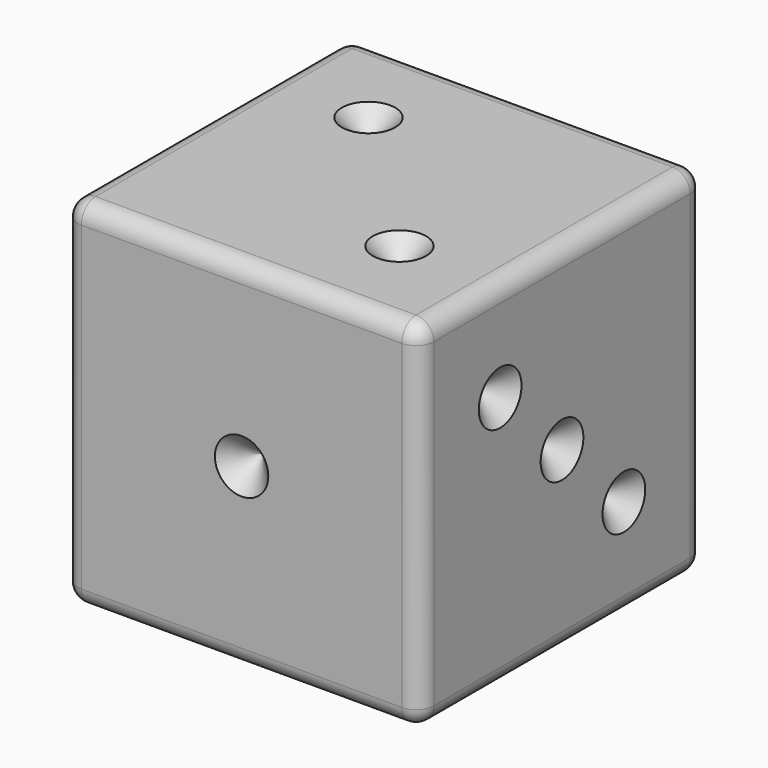
from build123d import *

# Parameters (mm, degrees)
F0_W      = 20
F0_H      = 20
F1_DEPTH  = 20
F2_R      = 1.5
F3_DEPTH  = 1.5
F4_R      = 1.5
F5_DEPTH  = 1.5
F6_R      = 1.5
F7_DEPTH  = 1.5
F8_R      = 1.5
F9_DEPTH  = 1.5
F10_R     = 1.5
F11_DEPTH = 1.5
F12_R     = 1.5
F13_DEPTH = 1.5
F14_R     = 1
F15_SIZE  = 1.49999


# Not quite as in the source:
# - a fillet or chamfer is up to 0.001 mm smaller than in the source, because OpenCascade refuses the exact size


with BuildPart() as f1:
    # F0 (on Top) → F1 (new body)
    with BuildSketch(Plane.XY):
        with Locations((10, 10)):
            Rectangle(F0_W, F0_H)
    extrude(amount=F1_DEPTH)

    # F2 (on face) → F3 (cut)
    with BuildSketch(Plane.XZ):
        with Locations((10, 10)):
            Circle(F2_R)
    extrude(amount=-F3_DEPTH, mode=Mode.SUBTRACT)

    # F4 (on face) → F5 (cut)
    with BuildSketch(Plane.XY.offset(20)):
        with Locations((14.3431457505, 5.6568542495)):
            Circle(F4_R)
        with Locations((5.6568542495, 14.3431457505)):
            Circle(F4_R)
    extrude(amount=-F5_DEPTH, mode=Mode.SUBTRACT)

    # F6 (on face) → F7 (cut)
    with BuildSketch(Plane.YZ.offset(20)):
        with Locations((5.6568542495, 14.3431457505)):
            Circle(F6_R)
        with Locations((10, 10)):
            Circle(F6_R)
        with Locations((14.3431457505, 5.6568542495)):
            Circle(F6_R)
    extrude(amount=-F7_DEPTH, mode=Mode.SUBTRACT)

    # F8 (on face) → F9 (cut)
    with BuildSketch(Plane(origin=(0, 20, 0), x_dir=(-1, 0, 0), z_dir=(0, 1, 0))):
        with Locations((-14.3431457505, 10)):
            Circle(F8_R)
        with Locations((-5.6568542495, 5.6568542495)):
            Circle(F8_R)
        with Locations((-14.3431457505, 14.3431457505)):
            Circle(F8_R)
        with Locations((-14.3431457505, 5.6568542495)):
            Circle(F8_R)
        with Locations((-5.6568542495, 14.3431457505)):
            Circle(F8_R)
        with Locations((-5.6568542495, 10)):
            Circle(F8_R)
    extrude(amount=-F9_DEPTH, mode=Mode.SUBTRACT)

    # F10 (on face) → F11 (cut)
    with BuildSketch(Plane(origin=(0, 0, 0), x_dir=(0, -1, 0), z_dir=(-1, 0, 0))):
        with Locations((-14.3431457505, 5.6568542495)):
            Circle(F10_R)
        with Locations((-5.6568542495, 5.6568542495)):
            Circle(F10_R)
        with Locations((-14.3431457505, 14.3431457505)):
            Circle(F10_R)
        with Locations((-5.6568542495, 14.3431457505)):
            Circle(F10_R)
    extrude(amount=-F11_DEPTH, mode=Mode.SUBTRACT)

    # F12 (on face) → F13 (cut)
    with BuildSketch(Plane(origin=(0, 0, 0), x_dir=(1, 0, 0), z_dir=(0, 0, -1))):
        with Locations((14.3431457505, -14.3431457505)):
            Circle(F12_R)
        with Locations((5.6568542495, -5.6568542495)):
            Circle(F12_R)
        with Locations((5.6568542495, -14.3431457505)):
            Circle(F12_R)
        with Locations((14.3431457505, -5.6568542495)):
            Circle(F12_R)
        with Locations((10, -10)):
            Circle(F12_R)
    extrude(amount=-F13_DEPTH, mode=Mode.SUBTRACT)

    # F14
    f14_edges = [f1.edges().sort_by_distance(p)[0] for p in [
        (20, 10, 20),
        (20, 0, 10),
        (10, 0, 20),
        (20, 20, 10),
        (20, 10, 0),
        (10, 20, 0),
        (0, 20, 10),
        (0, 10, 20),
        (10, 20, 20),
        (0, 0, 10),
        (0, 10, 0),
        (10, 0, 0),
    ]]
    fillet(f14_edges, radius=F14_R)

    # F15 (size 1.5 in the source; OpenCascade refuses exactly that, so slightly less here)
    f15_edges = [f1.edges().sort_by_distance(p)[0] for p in [
        (12.843146, 5.656854, 18.5),
        (8.5, 1.5, 10),
        (4.156854, 14.343146, 18.5),
        (15.843146, 18.5, 14.343146),
        (15.843146, 18.5, 10),
        (15.843146, 18.5, 5.656854),
        (7.156854, 18.5, 5.656854),
        (7.156854, 18.5, 10),
        (7.156854, 18.5, 14.343146),
        (18.5, 4.156854, 14.343146),
        (18.5, 8.5, 10),
        (18.5, 12.843146, 5.656854),
        (1.5, 15.843146, 14.343146),
        (1.5, 7.156854, 14.343146),
        (1.5, 7.156854, 5.656854),
        (1.5, 15.843146, 5.656854),
        (4.156854, 5.656854, 1.5),
        (4.156854, 14.343146, 1.5),
        (8.5, 10, 1.5),
        (12.843146, 14.343146, 1.5),
        (12.843146, 5.656854, 1.5),
    ]]
    chamfer(f15_edges, length=F15_SIZE)


solid = f1.part
